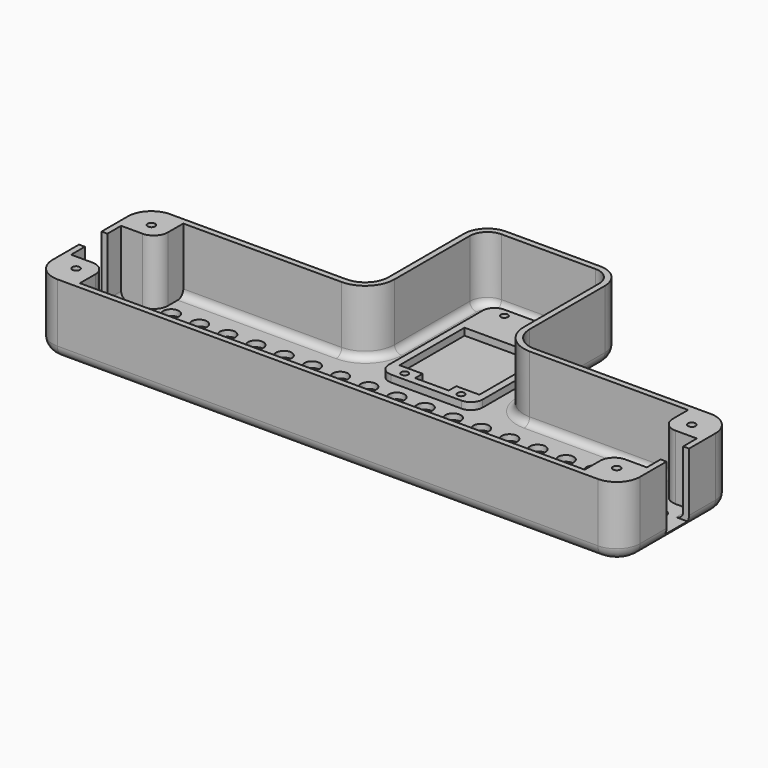
from build123d import *

# Parameters (mm, degrees)
F1_DEPTH      = 30
F2_R          = 10
F3_T          = -2.5
F4_W          = 40
F4_H          = 60
F5_DEPTH      = 3
F6_W          = 12
F6_H          = 27.5
F7_DEPTH      = 313
F8_R          = 3.2989534582
F9_DEPTH      = 25
F10_T1_DEPTH  = 75
F10_T3_DEPTH  = 40
F10_T5_DEPTH  = 40
F10_T7_DEPTH  = 75
F10_T9_DEPTH  = 40
F10_T11_DEPTH = 230
F10_T14_ANGLE = 90
F10_T16_ANGLE = 90
F10_T18_ANGLE = 90
F10_T20_ANGLE = 90
F10_T22_ANGLE = 90
F10_T24_ANGLE = 90
F10_T26_ANGLE = 90
F10_T28_ANGLE = 90
F11_R         = 3
F12_R         = 1.5019313846
F13_DEPTH     = 25
F15_DEPTH     = 3
F16_R         = 5
F17_R         = 3.2989534582
F18_DEPTH     = 2.5
F19_R         = 1.6
F20_DEPTH     = 27.5
F21_R         = 6


# Not quite as in the source:
# - a fillet or chamfer that OpenCascade refuses, or shapes differently, is made with other operations: its cross-section is extruded or revolved along the edge and cut away or added


with BuildPart() as f1:
    # F0 (on Top) → F1 (new body)
    with BuildSketch(Plane.XY):
        Polygon((-125, -30), (125, -30), (125, 30), (30, 30), (30, 90), (-30, 90), (-30, 30), (-125, 30), align=None)
    extrude(amount=F1_DEPTH)

    # F2
    f2_edges = [f1.edges().sort_by_distance(p)[0] for p in [
        (30, 30, 15),
        (-30, 30, 15),
        (-30, 90, 15),
        (30, 90, 15),
        (125, 30, 15),
        (125, -30, 15),
        (-125, -30, 15),
        (-125, 30, 15),
    ]]
    fillet(f2_edges, radius=F2_R)

    # F3
    f3_openings = [f1.faces().sort_by_distance(p)[0] for p in [
        (0, 11.538008, 30),
    ]]
    offset(amount=F3_T, openings=f3_openings)

    # F4 (on face) → F5 (join)
    with BuildSketch(Plane.XY.offset(2.5)):
        with Locations((0, 52.5)):
            Rectangle(F4_W, F4_H)
    extrude(amount=F5_DEPTH)

    # F6 (on face) → F7 (cut)
    with BuildSketch(Plane(origin=(-125, 0, 0), x_dir=(0, -1, 0), z_dir=(-1, 0, 0))):
        with Locations((0, 16.25)):
            Rectangle(F6_W, F6_H)
    extrude(amount=-F7_DEPTH, mode=Mode.SUBTRACT)

    # F8 (on face) → F9 (cut)
    with BuildSketch(Plane.XY.offset(2.5)):
        with Locations((-115, 15.5)):
            Circle(F8_R)
        with Locations((-115, 4.5)):
            Circle(F8_R)
        with Locations((-115, -17.5)):
            Circle(F8_R)
        with Locations((-115, -6.5)):
            Circle(F8_R)
        with Locations((-103, 4.5)):
            Circle(F8_R)
        with Locations((-103, 15.5)):
            Circle(F8_R)
        with Locations((-103, -17.5)):
            Circle(F8_R)
        with Locations((-103, -6.5)):
            Circle(F8_R)
        with Locations((-91, 4.5)):
            Circle(F8_R)
        with Locations((-91, 15.5)):
            Circle(F8_R)
        with Locations((-91, -17.5)):
            Circle(F8_R)
        with Locations((-91, -6.5)):
            Circle(F8_R)
        with Locations((-79, 4.5)):
            Circle(F8_R)
        with Locations((-79, 15.5)):
            Circle(F8_R)
        with Locations((-79, -17.5)):
            Circle(F8_R)
        with Locations((-79, -6.5)):
            Circle(F8_R)
        with Locations((-67, 4.5)):
            Circle(F8_R)
        with Locations((-67, 15.5)):
            Circle(F8_R)
        with Locations((-67, -17.5)):
            Circle(F8_R)
        with Locations((-67, -6.5)):
            Circle(F8_R)
        with Locations((-55, 4.5)):
            Circle(F8_R)
        with Locations((-55, 15.5)):
            Circle(F8_R)
        with Locations((-55, -17.5)):
            Circle(F8_R)
        with Locations((-55, -6.5)):
            Circle(F8_R)
        with Locations((-43, 4.5)):
            Circle(F8_R)
        with Locations((-43, 15.5)):
            Circle(F8_R)
        with Locations((-43, -17.5)):
            Circle(F8_R)
        with Locations((-43, -6.5)):
            Circle(F8_R)
        with Locations((-31, 4.5)):
            Circle(F8_R)
        with Locations((-31, 15.5)):
            Circle(F8_R)
        with Locations((-31, -17.5)):
            Circle(F8_R)
        with Locations((-31, -6.5)):
            Circle(F8_R)
        with Locations((-19, 4.5)):
            Circle(F8_R)
        with Locations((-19, 15.5)):
            Circle(F8_R)
        with Locations((-19, -17.5)):
            Circle(F8_R)
        with Locations((-19, -6.5)):
            Circle(F8_R)
        with Locations((-7, 4.5)):
            Circle(F8_R)
        with Locations((-7, 15.5)):
            Circle(F8_R)
        with Locations((-7, -17.5)):
            Circle(F8_R)
        with Locations((-7, -6.5)):
            Circle(F8_R)
        with Locations((5, 4.5)):
            Circle(F8_R)
        with Locations((5, 15.5)):
            Circle(F8_R)
        with Locations((5, -17.5)):
            Circle(F8_R)
        with Locations((5, -6.5)):
            Circle(F8_R)
        with Locations((17, 4.5)):
            Circle(F8_R)
        with Locations((17, 15.5)):
            Circle(F8_R)
        with Locations((17, -17.5)):
            Circle(F8_R)
        with Locations((17, -6.5)):
            Circle(F8_R)
        with Locations((29, 4.5)):
            Circle(F8_R)
        with Locations((29, 15.5)):
            Circle(F8_R)
        with Locations((29, -17.5)):
            Circle(F8_R)
        with Locations((29, -6.5)):
            Circle(F8_R)
        with Locations((41, 4.5)):
            Circle(F8_R)
        with Locations((41, 15.5)):
            Circle(F8_R)
        with Locations((41, -17.5)):
            Circle(F8_R)
        with Locations((41, -6.5)):
            Circle(F8_R)
        with Locations((53, 4.5)):
            Circle(F8_R)
        with Locations((53, 15.5)):
            Circle(F8_R)
        with Locations((53, -17.5)):
            Circle(F8_R)
        with Locations((53, -6.5)):
            Circle(F8_R)
        with Locations((65, 4.5)):
            Circle(F8_R)
        with Locations((65, 15.5)):
            Circle(F8_R)
        with Locations((65, -17.5)):
            Circle(F8_R)
        with Locations((65, -6.5)):
            Circle(F8_R)
        with Locations((77, 4.5)):
            Circle(F8_R)
        with Locations((77, 15.5)):
            Circle(F8_R)
        with Locations((77, -17.5)):
            Circle(F8_R)
        with Locations((77, -6.5)):
            Circle(F8_R)
        with Locations((89, 4.5)):
            Circle(F8_R)
        with Locations((89, 15.5)):
            Circle(F8_R)
        with Locations((89, -17.5)):
            Circle(F8_R)
        with Locations((89, -6.5)):
            Circle(F8_R)
        with Locations((101, 4.5)):
            Circle(F8_R)
        with Locations((101, 15.5)):
            Circle(F8_R)
        with Locations((101, -17.5)):
            Circle(F8_R)
        with Locations((101, -6.5)):
            Circle(F8_R)
        with Locations((113, 4.5)):
            Circle(F8_R)
        with Locations((113, 15.5)):
            Circle(F8_R)
        with Locations((113, -17.5)):
            Circle(F8_R)
        with Locations((113, -6.5)):
            Circle(F8_R)
    extrude(amount=-F9_DEPTH, mode=Mode.SUBTRACT)

    # F10: fillet of radius 5 on 1 edges, made by hand

    # F10_s2 → F10_t1 (cut)
    with BuildSketch(Plane.YZ.offset(40)):
        with BuildLine():
            ThreePointArc((25, 0), (28.5355339059, 1.4644660941), (30, 5))
            Line((30, 5), (30, 0))
            Line((30, 0), (25, 0))
        make_face()
    extrude(amount=F10_T1_DEPTH, mode=Mode.SUBTRACT)

    # F10_s4 → F10_t3 (cut)
    with BuildSketch(Plane.XZ.offset(-80)):
        with BuildLine():
            ThreePointArc((25, 0), (28.5355339059, 1.4644660941), (30, 5))
            Line((30, 5), (30, 0))
            Line((30, 0), (25, 0))
        make_face()
        with BuildLine():
            ThreePointArc((-25, 0), (-28.5355339059, 1.4644660941), (-30, 5))
            Line((-30, 5), (-30, 0))
            Line((-30, 0), (-25, 0))
        make_face()
    extrude(amount=F10_T3_DEPTH, mode=Mode.SUBTRACT)

    # F10_s6 → F10_t5 (cut)
    with BuildSketch(Plane.YZ.offset(-20)):
        with BuildLine():
            ThreePointArc((85, 0), (88.5355339059, 1.4644660941), (90, 5))
            Line((90, 5), (90, 0))
            Line((90, 0), (85, 0))
        make_face()
    extrude(amount=F10_T5_DEPTH, mode=Mode.SUBTRACT)

    # F10_s8 → F10_t7 (cut)
    with BuildSketch(Plane.YZ.offset(-115)):
        with BuildLine():
            ThreePointArc((25, 0), (28.5355339059, 1.4644660941), (30, 5))
            Line((30, 5), (30, 0))
            Line((30, 0), (25, 0))
        make_face()
    extrude(amount=F10_T7_DEPTH, mode=Mode.SUBTRACT)

    # F10_s10 → F10_t9 (cut)
    with BuildSketch(Plane.XZ.offset(-20)):
        with BuildLine():
            ThreePointArc((-120, 0), (-123.5355339059, 1.4644660941), (-125, 5))
            Line((-125, 5), (-125, 0))
            Line((-125, 0), (-120, 0))
        make_face()
        with BuildLine():
            ThreePointArc((120, 0), (123.5355339059, 1.4644660941), (125, 5))
            Line((125, 5), (125, 0))
            Line((125, 0), (120, 0))
        make_face()
    extrude(amount=F10_T9_DEPTH, mode=Mode.SUBTRACT)

    # F10_s12 → F10_t11 (cut)
    with BuildSketch(Plane.YZ.offset(-115)):
        with BuildLine():
            ThreePointArc((-30, 5), (-28.5355339059, 1.4644660941), (-25, 0))
            Line((-25, 0), (-30, 0))
            Line((-30, 0), (-30, 5))
        make_face()
    extrude(amount=F10_T11_DEPTH, mode=Mode.SUBTRACT)

    # F10_s13 → F10_t14 (revolve, cut)
    with BuildSketch(Plane.YZ.offset(40)):
        with BuildLine():
            ThreePointArc((25, 0), (28.5355339059, 1.4644660941), (30, 5))
            Line((30, 5), (30, 0))
            Line((30, 0), (25, 0))
        make_face()
    revolve(axis=Axis((40, 40, 0), (0, 0, -1)), revolution_arc=F10_T14_ANGLE, mode=Mode.SUBTRACT)

    # F10_s15 → F10_t16 (revolve, cut)
    with BuildSketch(Plane.XZ.offset(-80)):
        with BuildLine():
            ThreePointArc((25, 0), (28.5355339059, 1.4644660941), (30, 5))
            Line((30, 5), (30, 0))
            Line((30, 0), (25, 0))
        make_face()
    revolve(axis=Axis((20, 80, 0), (0, 0, 1)), revolution_arc=F10_T16_ANGLE, mode=Mode.SUBTRACT)

    # F10_s17 → F10_t18 (revolve, cut)
    with BuildSketch(Plane.YZ.offset(-20)):
        with BuildLine():
            ThreePointArc((85, 0), (88.5355339059, 1.4644660941), (90, 5))
            Line((90, 5), (90, 0))
            Line((90, 0), (85, 0))
        make_face()
    revolve(axis=Axis((-20, 80, 0), (0, 0, 1)), revolution_arc=F10_T18_ANGLE, mode=Mode.SUBTRACT)

    # F10_s19 → F10_t20 (revolve, cut)
    with BuildSketch(Plane.XZ.offset(-40)):
        with BuildLine():
            ThreePointArc((-25, 0), (-28.5355339059, 1.4644660941), (-30, 5))
            Line((-30, 5), (-30, 0))
            Line((-30, 0), (-25, 0))
        make_face()
    revolve(axis=Axis((-40, 40, 0), (0, 0, -1)), revolution_arc=F10_T20_ANGLE, mode=Mode.SUBTRACT)

    # F10_s21 → F10_t22 (revolve, cut)
    with BuildSketch(Plane.YZ.offset(-115)):
        with BuildLine():
            ThreePointArc((25, 0), (28.5355339059, 1.4644660941), (30, 5))
            Line((30, 5), (30, 0))
            Line((30, 0), (25, 0))
        make_face()
    revolve(axis=Axis((-115, 20, 0), (0, 0, 1)), revolution_arc=F10_T22_ANGLE, mode=Mode.SUBTRACT)

    # F10_s23 → F10_t24 (revolve, cut)
    with BuildSketch(Plane.YZ.offset(-115)):
        with BuildLine():
            ThreePointArc((-25, 0), (-28.5355339059, 1.4644660941), (-30, 5))
            Line((-30, 5), (-30, 0))
            Line((-30, 0), (-25, 0))
        make_face()
    revolve(axis=Axis((-115, -20, 0), (0, 0, -1)), revolution_arc=F10_T24_ANGLE, mode=Mode.SUBTRACT)

    # F10_s25 → F10_t26 (revolve, cut)
    with BuildSketch(Plane.YZ.offset(115)):
        with BuildLine():
            ThreePointArc((-25, 0), (-28.5355339059, 1.4644660941), (-30, 5))
            Line((-30, 5), (-30, 0))
            Line((-30, 0), (-25, 0))
        make_face()
    revolve(axis=Axis((115, -20, 0), (0, 0, 1)), revolution_arc=F10_T26_ANGLE, mode=Mode.SUBTRACT)

    # F10_s27 → F10_t28 (revolve, cut)
    with BuildSketch(Plane.XZ.offset(-20)):
        with BuildLine():
            ThreePointArc((120, 0), (123.5355339059, 1.4644660941), (125, 5))
            Line((125, 5), (125, 0))
            Line((125, 0), (120, 0))
        make_face()
    revolve(axis=Axis((115, 20, 0), (0, 0, 1)), revolution_arc=F10_T28_ANGLE, mode=Mode.SUBTRACT)

    # F11
    f11_edges = [f1.edges().sort_by_distance(p)[0] for p in [
        (-77.5, 27.5, 2.5),
        (0, -27.5, 2.5),
    ]]
    fillet(f11_edges, radius=F11_R)

    # F12 (on face) → F13 (cut)
    with BuildSketch(Plane.XY.offset(5.5)):
        with Locations((-12, 79)):
            Circle(F12_R)
        with Locations((12, 79)):
            Circle(F12_R)
        with Locations((-12, 26)):
            Circle(F12_R)
        with Locations((12, 26)):
            Circle(F12_R)
    extrude(amount=-F13_DEPTH, mode=Mode.SUBTRACT)

    # F14 (on face) → F15 (cut)
    with BuildSketch(Plane.XY.offset(5.5)):
        Polygon((17, 64.1045421362), (-17, 64.1045421362), (-17, 29.5), (-7.1533711464, 29.5), (-7.1533711464, 25.5), (7.1533711464, 25.5), (7.1533711464, 29.5), (17, 29.5), align=None)
    extrude(amount=-F15_DEPTH, mode=Mode.SUBTRACT)

    # F16
    f16_edges = [f1.edges().sort_by_distance(p)[0] for p in [
        (-20, 22.5, 4),
        (20, 22.5, 4),
        (-20, 82.5, 4),
        (20, 82.5, 4),
    ]]
    fillet(f16_edges, radius=F16_R)

    # F17 (on face) → F18 (join, through all)
    with BuildSketch(Plane.XY.offset(2.5)):
        with Locations((-115, 15.5)):
            Circle(F17_R)
        with Locations((113, 15.5)):
            Circle(F17_R)
        with Locations((113, -17.5)):
            Circle(F17_R)
        with Locations((-115, -17.5)):
            Circle(F17_R)
    extrude(amount=-F18_DEPTH)

    # F19 (on face) → F20 (join, through all)
    with BuildSketch(Plane.XY.offset(30)):
        with BuildLine():
            Line((-107.4046194553, 13.3073404431), (-107.4046194553, 27.5))
            Line((-107.4046194553, 27.5), (-115, 27.5))
            ThreePointArc((-115, 27.5), (-120.3033008589, 25.3033008589), (-122.5, 20))
            Line((-122.5, 20), (-122.5, 13.3073404431))
            Line((-122.5, 13.3073404431), (-107.4046194553, 13.3073404431))
        make_face()
        with Locations((-115, 20)):
            Circle(F19_R, mode=Mode.SUBTRACT)
        with BuildLine():
            Line((-115, -27.5), (-107.4046194553, -27.5))
            Line((-107.4046194553, -27.5), (-107.4046194553, -13.3073404431))
            Line((-107.4046194553, -13.3073404431), (-122.5, -13.3073404431))
            Line((-122.5, -13.3073404431), (-122.5, -20))
            ThreePointArc((-122.5, -20), (-120.3033008589, -25.3033008589), (-115, -27.5))
        make_face()
        with Locations((-115, -20)):
            Circle(F19_R, mode=Mode.SUBTRACT)
        with BuildLine():
            Line((107.4046194553, -13.3073404431), (107.4046194553, -27.5))
            Line((107.4046194553, -27.5), (115, -27.5))
            ThreePointArc((115, -27.5), (120.3033008589, -25.3033008589), (122.5, -20))
            Line((122.5, -20), (122.5, -13.3073404431))
            Line((122.5, -13.3073404431), (107.4046194553, -13.3073404431))
        make_face()
        with Locations((115, -20)):
            Circle(F19_R, mode=Mode.SUBTRACT)
        with BuildLine():
            Line((115, 27.5), (107.4046194553, 27.5))
            Line((107.4046194553, 27.5), (107.4046194553, 13.3073404431))
            Line((107.4046194553, 13.3073404431), (122.5, 13.3073404431))
            Line((122.5, 13.3073404431), (122.5, 20))
            ThreePointArc((122.5, 20), (120.3033008589, 25.3033008589), (115, 27.5))
        make_face()
        with Locations((115, 20)):
            Circle(F19_R, mode=Mode.SUBTRACT)
    extrude(amount=-F20_DEPTH)

    # F21
    f21_edges = [f1.edges().sort_by_distance(p)[0] for p in [
        (-107.404619, 13.30734, 16.25),
        (107.404619, 13.30734, 16.25),
        (107.404619, -13.30734, 16.25),
        (-107.404619, -13.30734, 16.25),
    ]]
    fillet(f21_edges, radius=F21_R)


solid = f1.part
